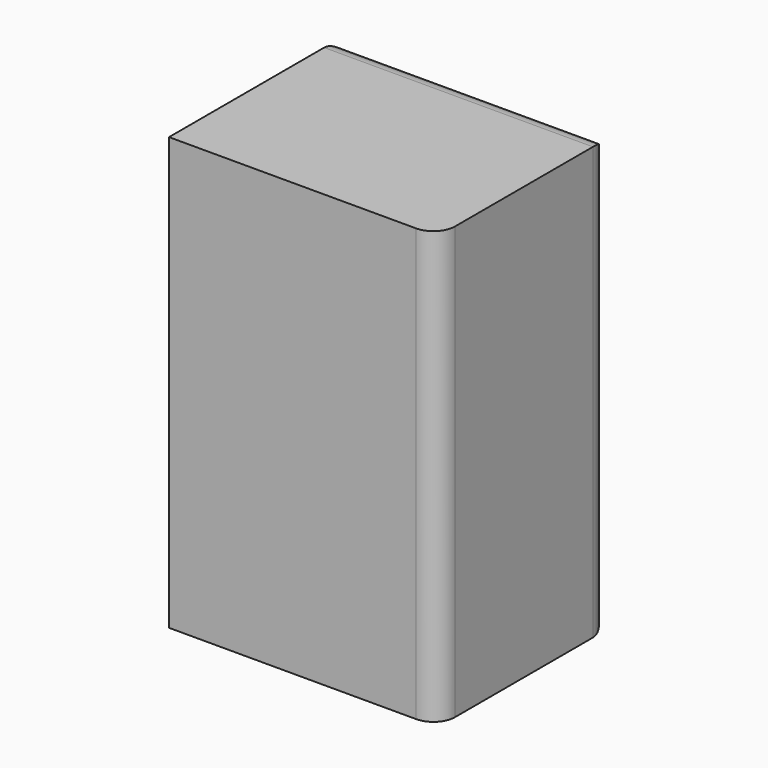
from build123d import *

# Parameters (mm, degrees)
F0_W        = 63.2100254297
F0_H        = 50.6872721016
F1_DEPTH    = 101.6
F2_T        = -3.048
F3_T1_DEPTH = 127
F3_T3_DEPTH = 88.6100254297


# Not quite as in the source:
# - a fillet or chamfer that OpenCascade refuses, or shapes differently, is made with other operations: its cross-section is extruded or revolved along the edge and cut away or added


with BuildPart() as f1:
    # F0 (on Top) → F1 (new body)
    with BuildSketch(Plane.XY):
        with Locations((31.6050127149, -25.3436360508)):
            Rectangle(F0_W, F0_H)
    extrude(amount=F1_DEPTH)

    # F2
    f2_openings = [f1.faces().sort_by_distance(p)[0] for p in [
        (31.605013, 0, 50.8),
    ]]
    offset(amount=F2_T, openings=f2_openings)

    # F3: fillet of radius 5.08 on 5 edges, made by hand

    # F3_s2 → F3_t1 (cut)
    with BuildSketch(Plane.XY.offset(-12.7)):
        with BuildLine():
            ThreePointArc((0, -5.08), (1.4878975516, -1.4878975516), (5.08, 0))
            Line((5.08, 0), (0, 0))
            Line((0, 0), (0, -5.08))
        make_face()
        with BuildLine():
            ThreePointArc((63.2100254297, -5.08), (61.7221278782, -1.4878975516), (58.1300254297, 0))
            Line((58.1300254297, 0), (63.2100254297, 0))
            Line((63.2100254297, 0), (63.2100254297, -5.08))
        make_face()
        with BuildLine():
            ThreePointArc((58.1300254297, -50.6872721016), (61.7221278782, -49.1993745501), (63.2100254297, -45.6072721016))
            Line((63.2100254297, -45.6072721016), (63.2100254297, -50.6872721016))
            Line((63.2100254297, -50.6872721016), (58.1300254297, -50.6872721016))
        make_face()
    extrude(amount=F3_T1_DEPTH, mode=Mode.SUBTRACT)

    # F3_s4 → F3_t3 (cut)
    with BuildSketch(Plane.YZ.offset(-12.7)):
        with BuildLine():
            ThreePointArc((-5.08, 101.6), (-1.4878975516, 100.1121024484), (0, 96.52))
            Line((0, 96.52), (0, 101.6))
            Line((0, 101.6), (-5.08, 101.6))
        make_face()
        with BuildLine():
            ThreePointArc((-5.08, 0), (-1.4878975516, 1.4878975516), (0, 5.08))
            Line((0, 5.08), (0, 0))
            Line((0, 0), (-5.08, 0))
        make_face()
    extrude(amount=F3_T3_DEPTH, mode=Mode.SUBTRACT)


solid = f1.part
